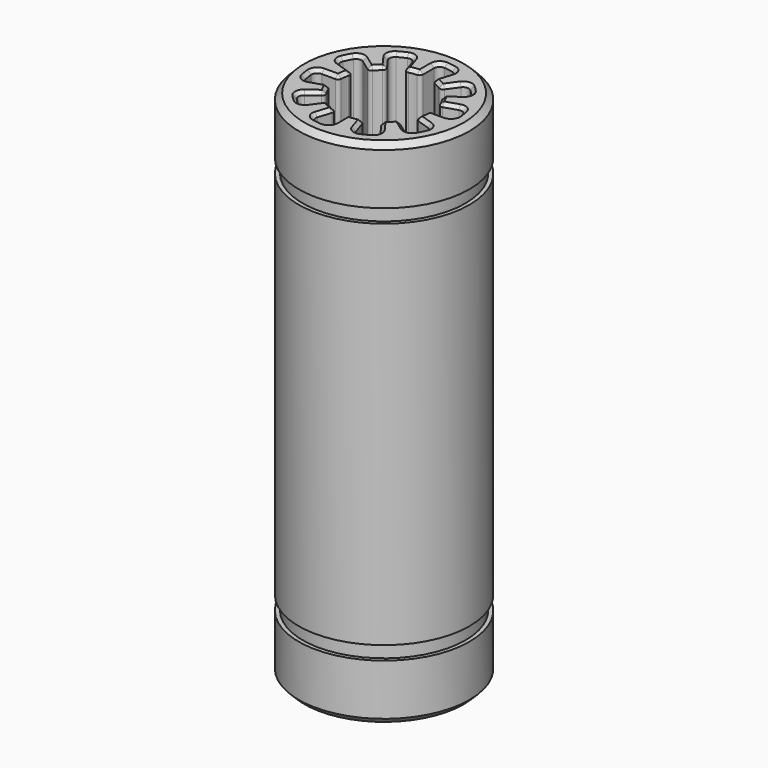
from build123d import *

# Parameters (mm, degrees)
F0_R     = 7.5
F1_DEPTH = 45
F3_R     = 8
F3_R_2   = 7.15
F4_DEPTH = 1.2
F6_R     = 8
F6_R_2   = 7.15
F7_DEPTH = 1.2
F8_SIZE  = 0.5
F9_R     = 0.3
F10_R    = 0.5
F11_SIZE = 0.29999


# Not quite as in the source:
# - a fillet or chamfer is up to 0.001 mm smaller than in the source, because OpenCascade refuses the exact size
# - a feature names something its author has since deleted; it is built from what else it names


with BuildPart() as f1:
    # F0 (on Top) → F1 (new body)
    with BuildSketch(Plane.XY):
        Circle(F0_R)
        with BuildLine():
            ThreePointArc((1.2360679775, 3.8042260652), (1.815961999, 3.5640260968), (2.3511410092, 3.2360679775))
            Line((2.3511410092, 3.2360679775), (3.5267115138, 4.8541019662))
            ThreePointArc((3.5267115138, 4.8541019662), (4.2426406871, 4.2426406871), (4.8541019662, 3.5267115138))
            Line((4.8541019662, 3.5267115138), (3.2360679775, 2.3511410092))
            ThreePointArc((3.2360679775, 2.3511410092), (3.5640260968, 1.815961999), (3.8042260652, 1.2360679775))
            Line((3.8042260652, 1.2360679775), (5.7063390978, 1.8541019662))
            ThreePointArc((5.7063390978, 1.8541019662), (5.9261300436, 0.9386067902), (6, 0))
            Line((6, 0), (4, 0))
            ThreePointArc((4, 0), (3.9507533624, -0.6257378602), (3.8042260652, -1.2360679775))
            Line((3.8042260652, -1.2360679775), (5.7063390978, -1.8541019662))
            ThreePointArc((5.7063390978, -1.8541019662), (5.3460391451, -2.7239429984), (4.8541019662, -3.5267115138))
            Line((4.8541019662, -3.5267115138), (3.2360679775, -2.3511410092))
            ThreePointArc((3.2360679775, -2.3511410092), (2.8284271247, -2.8284271247), (2.3511410092, -3.2360679775))
            Line((2.3511410092, -3.2360679775), (3.5267115138, -4.8541019662))
            ThreePointArc((3.5267115138, -4.8541019662), (2.7239429984, -5.3460391451), (1.8541019662, -5.7063390978))
            Line((1.8541019662, -5.7063390978), (1.2360679775, -3.8042260652))
            ThreePointArc((1.2360679775, -3.8042260652), (0.6257378602, -3.9507533624), (0, -4))
            Line((0, -4), (0, -6))
            ThreePointArc((0, -6), (-0.9386067902, -5.9261300436), (-1.8541019662, -5.7063390978))
            Line((-1.8541019662, -5.7063390978), (-1.2360679775, -3.8042260652))
            ThreePointArc((-1.2360679775, -3.8042260652), (-1.815961999, -3.5640260968), (-2.3511410092, -3.2360679775))
            Line((-2.3511410092, -3.2360679775), (-3.5267115138, -4.8541019662))
            ThreePointArc((-3.5267115138, -4.8541019662), (-4.2426406871, -4.2426406871), (-4.8541019662, -3.5267115138))
            Line((-4.8541019662, -3.5267115138), (-3.2360679775, -2.3511410092))
            ThreePointArc((-3.2360679775, -2.3511410092), (-3.5640260968, -1.815961999), (-3.8042260652, -1.2360679775))
            Line((-3.8042260652, -1.2360679775), (-5.7063390978, -1.8541019662))
            ThreePointArc((-5.7063390978, -1.8541019662), (-5.9261300436, -0.9386067902), (-6, 0))
            Line((-6, 0), (-4, 0))
            ThreePointArc((-4, 0), (-3.9507533624, 0.6257378602), (-3.8042260652, 1.2360679775))
            Line((-3.8042260652, 1.2360679775), (-5.7063390978, 1.8541019662))
            ThreePointArc((-5.7063390978, 1.8541019662), (-5.3460391451, 2.7239429984), (-4.8541019662, 3.5267115138))
            Line((-4.8541019662, 3.5267115138), (-3.2360679775, 2.3511410092))
            ThreePointArc((-3.2360679775, 2.3511410092), (-2.8284271247, 2.8284271247), (-2.3511410092, 3.2360679775))
            Line((-2.3511410092, 3.2360679775), (-3.5267115138, 4.8541019662))
            ThreePointArc((-3.5267115138, 4.8541019662), (-2.7239429984, 5.3460391451), (-1.8541019662, 5.7063390978))
            Line((-1.8541019662, 5.7063390978), (-1.2360679775, 3.8042260652))
            ThreePointArc((-1.2360679775, 3.8042260652), (-0.6257378602, 3.9507533624), (0, 4))
            Line((0, 4), (0, 6))
            ThreePointArc((0, 6), (0.9386067902, 5.9261300436), (1.8541019662, 5.7063390978))
            Line((1.8541019662, 5.7063390978), (1.2360679775, 3.8042260652))
        make_face(mode=Mode.SUBTRACT)
    extrude(amount=F1_DEPTH)

    # F3 (on offset) → F4 (cut)
    with BuildSketch(Plane.XY.offset(5)):
        Circle(F3_R)
        Circle(F3_R_2, mode=Mode.SUBTRACT)
    extrude(amount=F4_DEPTH, mode=Mode.SUBTRACT)

    # F6 (on offset) → F7 (cut)
    with BuildSketch(Plane.XY.offset(40)):
        Circle(F6_R)
        Circle(F6_R_2, mode=Mode.SUBTRACT)
    extrude(amount=-F7_DEPTH, mode=Mode.SUBTRACT)

    # F8
    f8_edges = [f1.edges().sort_by_distance(p)[0] for p in [
        (-7.5, 0, 45),
        (-7.5, 0, 0),
    ]]
    chamfer(f8_edges, length=F8_SIZE)

    # F9
    f9_edges = [f1.edges().sort_by_distance(p)[0] for p in [
        (2.351141, 3.236068, 22.5),
        (1.236068, 3.804226, 22.5),
        (3.236068, 2.351141, 22.5),
        (3.804226, 1.236068, 22.5),
        (4, 0, 22.5),
        (3.804226, -1.236068, 22.5),
        (3.236068, -2.351141, 22.5),
        (2.351141, -3.236068, 22.5),
        (1.236068, -3.804226, 22.5),
        (0, -4, 22.5),
        (-1.236068, -3.804226, 22.5),
        (-2.351141, -3.236068, 22.5),
        (-3.236068, -2.351141, 22.5),
        (-3.804226, -1.236068, 22.5),
        (-4, 0, 22.5),
        (-3.804226, 1.236068, 22.5),
        (-3.236068, 2.351141, 22.5),
        (-2.351141, 3.236068, 22.5),
        (-1.236068, 3.804226, 22.5),
        (0, 4, 22.5),
    ]]
    fillet(f9_edges, radius=F9_R)

    # F10
    f10_edges = [f1.edges().sort_by_distance(p)[0] for p in [
        (0, 6, 22.5),
        (1.854102, 5.706339, 22.5),
        (4.854102, 3.526712, 22.5),
        (5.706339, 1.854102, 22.5),
        (6, 0, 22.5),
        (5.706339, -1.854102, 22.5),
        (4.854102, -3.526712, 22.5),
        (3.526712, -4.854102, 22.5),
        (1.854102, -5.706339, 22.5),
        (-1.854102, -5.706339, 22.5),
        (0, -6, 22.5),
        (-3.526712, -4.854102, 22.5),
        (-4.854102, -3.526712, 22.5),
        (-5.706339, -1.854102, 22.5),
        (-6, 0, 22.5),
        (-5.706339, 1.854102, 22.5),
        (-4.854102, 3.526712, 22.5),
        (-3.526712, 4.854102, 22.5),
        (-1.854102, 5.706339, 22.5),
        (3.526712, 4.854102, 22.5),
    ]]
    fillet(f10_edges, radius=F10_R)

    # F11 (size 0.3 in the source; OpenCascade refuses exactly that, so slightly less here)
    f11_edges = [f1.edges().sort_by_distance(p)[0] for p in [
        (-3.950732, 2.870375, 45),
        (1.509046, 4.644365, 0),
        (1.651741, 5.610691, 0),
        (1.338959, 3.860089, 0),
        (0.938607, 5.92613, 0),
        (1.815962, 3.564026, 0),
        (0.1629, 5.8465, 0),
        (2.335857, 3.352144, 0),
        (0, 4.883374, 0),
        (2.870375, 3.950732, 0),
        (-0.080593, 4.084924, 0),
        (3.568275, 4.634168, 0),
        (-0.625738, 3.950753, 0),
        (4.242641, 4.242641, 0),
        (-1.185663, 3.909898, 0),
        (4.634168, 3.568275, 0),
        (-1.509046, 4.644365, 0),
        (3.950732, 2.870375, 0),
        (-1.961595, 5.510013, 0),
        (3.352144, 2.335857, 0),
        (-2.723943, 5.346039, 0),
        (3.564026, 1.815962, 0),
        (-3.304698, 4.825668, 0),
        (3.860089, 1.338959, 0),
        (-2.870375, 3.950732, 0),
        (4.644365, 1.509046, 0),
        (-2.466259, 3.257402, 0),
        (5.610691, 1.651741, 0),
        (-2.828427, 2.828427, 0),
        (5.92613, 0.938607, 0),
        (-3.257402, 2.466259, 0),
        (5.8465, 0.1629, 0),
        (-3.950732, 2.870375, 0),
        (4.883374, 0, 0),
        (-4.825668, 3.304698, 0),
        (4.084924, -0.080593, 0),
        (-5.346039, 2.723943, 0),
        (3.950753, -0.625738, 0),
        (-5.510013, 1.961595, 0),
        (3.909898, -1.185663, 0),
        (-4.644365, 1.509046, 0),
        (4.644365, -1.509046, 0),
        (-3.909898, 1.185663, 0),
        (5.510013, -1.961595, 0),
        (-3.950753, 0.625738, 0),
        (5.346039, -2.723943, 0),
        (-4.084924, 0.080593, 0),
        (4.825668, -3.304698, 0),
        (-4.883374, 0, 0),
        (3.950732, -2.870375, 0),
        (-5.8465, -0.1629, 0),
        (3.257402, -2.466259, 0),
        (-5.92613, -0.938607, 0),
        (2.828427, -2.828427, 0),
        (-5.610691, -1.651741, 0),
        (2.466259, -3.257402, 0),
        (-4.644365, -1.509046, 0),
        (2.870375, -3.950732, 0),
        (-3.860089, -1.338959, 0),
        (3.304698, -4.825668, 0),
        (-3.564026, -1.815962, 0),
        (2.723943, -5.346039, 0),
        (-3.352144, -2.335857, 0),
        (1.961595, -5.510013, 0),
        (-3.950732, -2.870375, 0),
        (1.509046, -4.644365, 0),
        (-4.634168, -3.568275, 0),
        (1.185663, -3.909898, 0),
        (-4.242641, -4.242641, 0),
        (0.625738, -3.950753, 0),
        (-3.568275, -4.634168, 0),
        (0.080593, -4.084924, 0),
        (-2.870375, -3.950732, 0),
        (0, -4.883374, 0),
        (-2.335857, -3.352144, 0),
        (-0.1629, -5.8465, 0),
        (-1.815962, -3.564026, 0),
        (-0.938607, -5.92613, 0),
        (-1.338959, -3.860089, 0),
        (-1.651741, -5.610691, 0),
        (-1.509046, -4.644365, 0),
        (1.509046, 4.644365, 45),
        (1.651741, 5.610691, 45),
        (1.338959, 3.860089, 45),
        (0.938607, 5.92613, 45),
        (1.815962, 3.564026, 45),
        (0.1629, 5.8465, 45),
        (2.335857, 3.352144, 45),
        (0, 4.883374, 45),
        (2.870375, 3.950732, 45),
        (-0.080593, 4.084924, 45),
        (3.568275, 4.634168, 45),
        (-0.625738, 3.950753, 45),
        (4.242641, 4.242641, 45),
        (-1.185663, 3.909898, 45),
        (4.634168, 3.568275, 45),
        (-1.509046, 4.644365, 45),
        (3.950732, 2.870375, 45),
        (-1.961595, 5.510013, 45),
        (3.352144, 2.335857, 45),
        (-2.723943, 5.346039, 45),
        (3.564026, 1.815962, 45),
        (-3.304698, 4.825668, 45),
        (3.860089, 1.338959, 45),
        (-2.870375, 3.950732, 45),
        (4.644365, 1.509046, 45),
        (-2.466259, 3.257402, 45),
        (5.610691, 1.651741, 45),
        (-2.828427, 2.828427, 45),
        (5.92613, 0.938607, 45),
        (-3.257402, 2.466259, 45),
        (5.8465, 0.1629, 45),
        (4.883374, 0, 45),
        (-4.825668, 3.304698, 45),
        (4.084924, -0.080593, 45),
        (-5.346039, 2.723943, 45),
        (3.950753, -0.625738, 45),
        (-5.510013, 1.961595, 45),
        (3.909898, -1.185663, 45),
        (-4.644365, 1.509046, 45),
        (4.644365, -1.509046, 45),
        (-3.909898, 1.185663, 45),
        (5.510013, -1.961595, 45),
        (-3.950753, 0.625738, 45),
        (5.346039, -2.723943, 45),
        (-4.084924, 0.080593, 45),
        (4.825668, -3.304698, 45),
        (-4.883374, 0, 45),
        (3.950732, -2.870375, 45),
        (-5.8465, -0.1629, 45),
        (3.257402, -2.466259, 45),
        (-5.92613, -0.938607, 45),
        (2.828427, -2.828427, 45),
        (-5.610691, -1.651741, 45),
        (2.466259, -3.257402, 45),
        (-4.644365, -1.509046, 45),
        (2.870375, -3.950732, 45),
        (-3.860089, -1.338959, 45),
        (3.304698, -4.825668, 45),
        (-3.564026, -1.815962, 45),
        (2.723943, -5.346039, 45),
        (-3.352144, -2.335857, 45),
        (1.961595, -5.510013, 45),
        (-3.950732, -2.870375, 45),
        (1.509046, -4.644365, 45),
        (-4.634168, -3.568275, 45),
        (1.185663, -3.909898, 45),
        (-4.242641, -4.242641, 45),
        (0.625738, -3.950753, 45),
        (-3.568275, -4.634168, 45),
        (0.080593, -4.084924, 45),
        (-2.870375, -3.950732, 45),
        (0, -4.883374, 45),
        (-2.335857, -3.352144, 45),
        (-0.1629, -5.8465, 45),
        (-1.815962, -3.564026, 45),
        (-0.938607, -5.92613, 45),
        (-1.338959, -3.860089, 45),
        (-1.651741, -5.610691, 45),
        (-1.509046, -4.644365, 45),
    ]]
    chamfer(f11_edges, length=F11_SIZE)


solid = f1.part
